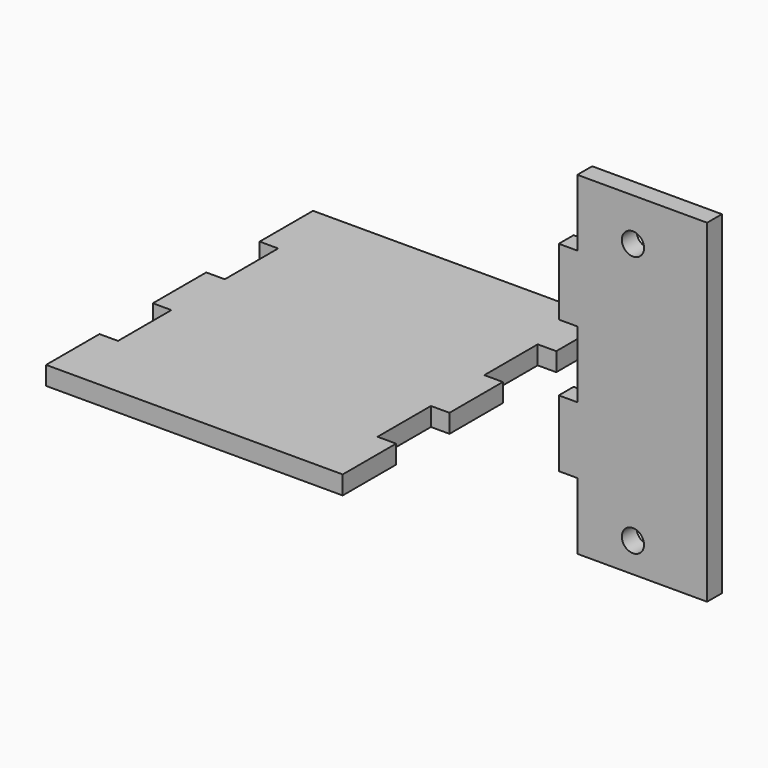
from build123d import *

# Parameters (mm, degrees)
F0_W     = 6.35
F0_H     = 22.86
F1_DEPTH = 6.35
F2_W     = 6.35
F2_H     = 22.86
F2_R     = 3.81
F3_DEPTH = 6.35


# Not quite as in the source:
# - a length typed as a fraction of an inch, garbled in the dataset ("3 / 203.2 mm" for 3/8 in), is restored


with BuildPart() as f1:
    # F0 (on Top) → F1 (new body)
    with BuildSketch(Plane.XY):
        with Locations((-20.988421008, 30.6906817461)):
            Rectangle(F0_W, F0_H)
        with Locations((-20.988421008, -60.7493182539)):
            Rectangle(F0_W, F0_H)
        Polygon((-24.163421008, 42.1206817461), (-68.613421008, 42.1206817461), (-119.413421008, 42.1206817461), (-119.413421008, 19.2606817461), (-113.063421008, 19.2606817461), (-113.063421008, -3.5993182539), (-119.413421008, -3.5993182539), (-119.413421008, -26.4593182539), (-113.063421008, -26.4593182539), (-113.063421008, -49.3193182539), (-119.413421008, -49.3193182539), (-119.413421008, -72.1793182539), (-68.613421008, -72.1793182539), (-24.163421008, -72.1793182539), (-24.163421008, -49.3193182539), (-24.163421008, -26.4593182539), (-24.163421008, -3.5993182539), (-24.163421008, 19.2606817461), align=None)
        with Locations((-20.988421008, -15.0293182539)):
            Rectangle(F0_W, F0_H)
    extrude(amount=F1_DEPTH)


with BuildPart() as f3:
    # F2 (on Front) → F3 (new body)
    with BuildSketch(Plane.XZ):
        with Locations((6.7176349759, 44.6672367319)):
            Rectangle(F2_W, F2_H)
        with Locations((6.7176349759, -1.0527632681)):
            Rectangle(F2_W, F2_H)
        Polygon((54.3426349759, 78.9572367319), (9.8926349759, 78.9572367319), (9.8926349759, 56.0972367319), (9.8926349759, 33.2372367319), (9.8926349759, 10.3772367319), (9.8926349759, -12.4827632681), (9.8926349759, -35.3427632681), (54.3426349759, -35.3427632681), align=None)
        with Locations((28.9426349759, -25.1827632681)):
            Circle(F2_R, mode=Mode.SUBTRACT)
        with Locations((28.9426349759, 64.3128305674)):
            Circle(F2_R, mode=Mode.SUBTRACT)
    extrude(amount=F3_DEPTH)


solid = Compound([f1.part, f3.part])
